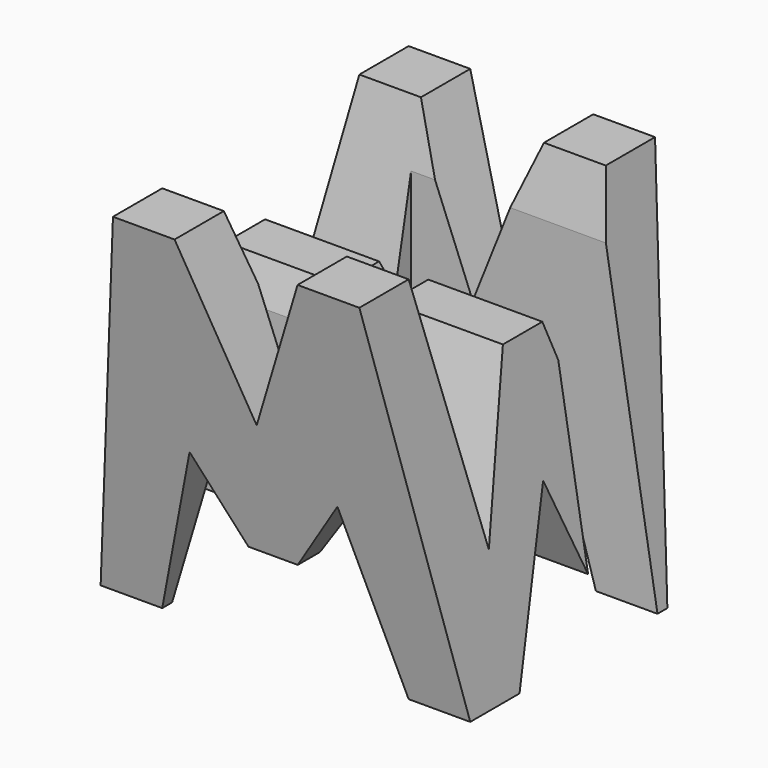
from build123d import *

# Parameters (mm, degrees)
F0_W      = 38.1
F0_H      = 38.099996
F1_DEPTH  = 38.1
F6_DEPTH  = 38.1
F8_DEPTH  = 38.1
F9_W      = 25.4
F9_H      = 7.62
F10_DEPTH = 38.1


# Not quite as in the source:
# - ends of sketch curves that miss each other by under 0.0002 mm in the source are joined


with BuildPart() as f1:
    # F0 (on Front) → F1 (new body)
    with BuildSketch(Plane.XZ):
        with Locations((19.05, 19.049998)):
            Rectangle(F0_W, F0_H)
    extrude(amount=F1_DEPTH)

    # F5 (on offset) → F6 (cut)
    with BuildSketch(Plane.YZ.offset(38.1)):
        Polygon((0, 0), (0, 38.099999), (-6.35, 0), align=None)
        Polygon((-11.43, 13.398314), (-6.35, 38.099999), (-31.75, 38.1), (-26.67, 12.888374), (-21.59, 28.575), (-16.51, 28.575), align=None)
        Polygon((-25.4, 0), (-12.7, 0), (-19.05, 15.875), align=None)
        Polygon((-31.75, 0), (-38.1, 38.1), (-38.1, 0), align=None)
    extrude(amount=-F6_DEPTH, mode=Mode.SUBTRACT)

    # F7 (on offset) → F8 (cut)
    with BuildSketch(Plane.XZ.offset(38.1)):
        Polygon((0, 38.100007), (0, 0), (6.35, 38.1), align=None)
        Polygon((25.4, 38.154688), (12.7, 38.1), (19.05, 22.225), align=None)
        Polygon((31.75, 38.1), (38.1, 0), (38.1, 38.100007), align=None)
        Polygon((11.43, 16.971819), (6.35, 0), (31.75, 0), (26.67, 16.971819), (21.59, 9.525), (16.51, 9.525), align=None)
    extrude(amount=-F8_DEPTH, mode=Mode.SUBTRACT)

    # F9 (on offset) → F10 (cut)
    with BuildSketch(Plane.XY.offset(38.1)):
        with Locations((25.4, -11.43)):
            Rectangle(F9_W, F9_H)
        with Locations((12.7, -26.67)):
            Rectangle(F9_W, F9_H)
    extrude(amount=-F10_DEPTH, mode=Mode.SUBTRACT)


solid = f1.part
